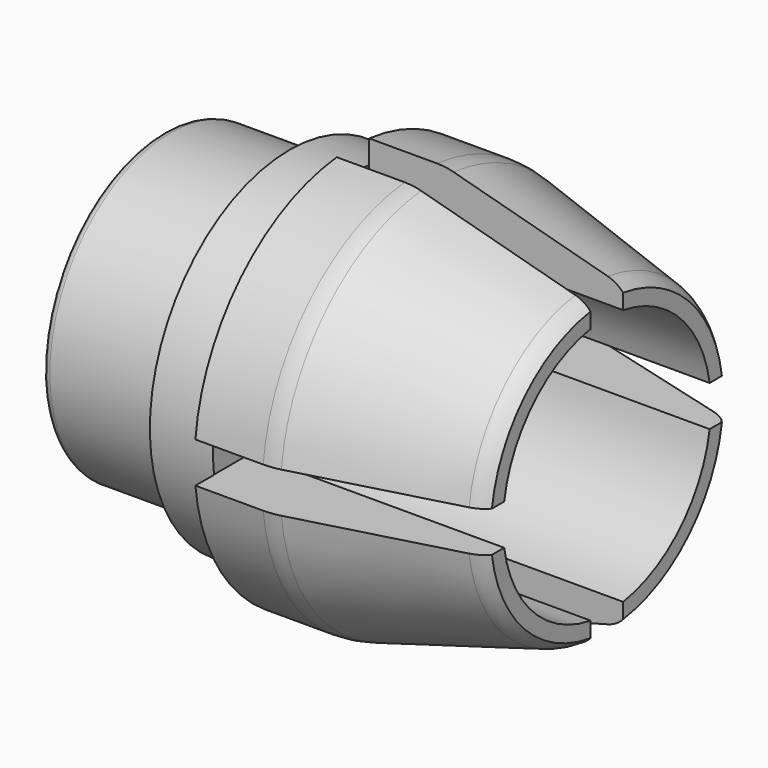
from build123d import *

# Parameters (mm, degrees)
F2_W          = 2.032
F2_H          = 3.556
F2_W_2        = 3.556
F2_H_2        = 2.032
F3_DEPTH      = 25.4
F3_DEPTH_BACK = 4.3434


# Not quite as in the source:
# - a feature names something its author has since deleted; it is built from what else it names


with BuildPart() as f1:
    # F0 (on Front) → F1 (revolve)
    with BuildSketch(Plane.XZ):
        with BuildLine():
            ThreePointArc((8.3732076521, 7.2620277332), (8.0243377529, 7.5505761386), (7.608205325, 7.728913435))
            Line((7.608205325, 7.728913435), (-0.1130385595, 9.7978144985))
            ThreePointArc((-0.1130385595, 9.7978144985), (-0.5203683675, 9.8788374349), (-0.9347890277, 9.906))
            Line((-0.9347890277, 9.906), (-4.3267923479, 9.906))
            Line((-4.3267923479, 9.906), (-4.3267923479, 8.73125))
            Line((-4.3267923479, 8.73125), (-7.5017923479, 8.73125))
            Line((-7.5017923479, 8.73125), (-7.5017923479, 7.5438))
            Line((-7.5017923479, 7.5438), (-13.4549173479, 7.5438))
            ThreePointArc((-13.4549173479, 7.5438), (-13.7355503517, 7.4275580038), (-13.8517923479, 7.146925))
            Line((-13.8517923479, 7.146925), (-13.8517923479, 6.5024))
            Line((-13.8517923479, 6.5024), (8.3732076521, 6.5024))
            Line((8.3732076521, 6.5024), (8.3732076521, 7.2620277332))
        make_face()
    revolve(axis=Axis((-0.2325048039, 0, 0), (1, 0, 0)))

    # F2 (on Right) → F3 (cut, two sides)
    with BuildSketch(Plane.YZ) as f3_sk:
        with Locations((0, -8.1534)):
            Rectangle(F2_W, F2_H)
        with Locations((0, 8.1534)):
            Rectangle(F2_W, F2_H)
        with Locations((-8.1534, 0)):
            Rectangle(F2_W_2, F2_H_2)
        with Locations((8.1534, 0)):
            Rectangle(F2_W_2, F2_H_2)
    extrude(amount=F3_DEPTH, mode=Mode.SUBTRACT)
    extrude(f3_sk.sketch, amount=-F3_DEPTH_BACK, mode=Mode.SUBTRACT)


solid = f1.part
